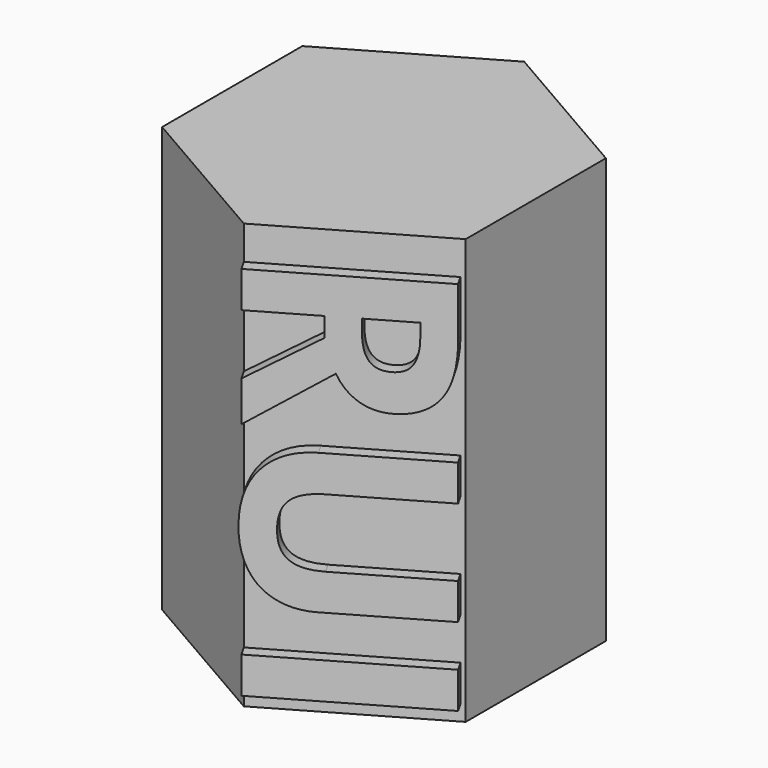
from build123d import *

# Parameters (mm, degrees)
F1_DEPTH     = 350
F3_TEXT_SIZE = 197.4233351479
F4_DEPTH     = 10
F6_DEPTH     = 300
F7_R         = 15


# Not quite as in the source:
# - Text() gives the source's letters only with a copy of the font that has no kerning and outlines rounded to 1/6400 em; it was checked with that copy


with BuildPart() as f1:
    # F0 (on Top) → F1 (new body)
    with BuildSketch(Plane.XY):
        Polygon((125, -72.1687836487), (125, 72.1687836487), (0, 144.3375672974), (-125, 72.1687836487), (-125, -72.1687836487), (0, -144.3375672974), align=None)
    extrude(amount=F1_DEPTH)

    # F3 (on face) → F4 (join)
    with BuildSketch(Plane(origin=(62.5, -108.2531754731, 0), x_dir=(0.8660254038, 0.5, 0), z_dir=(0.5, -0.8660254038, 0))):
        with Locations(Location((-72.1687836487, 340), (0, 0, -90))):
            Text('RUI', F3_TEXT_SIZE, font='Open Sans', font_style=FontStyle.BOLD, text_align=(TextAlign.LEFT, TextAlign.BOTTOM))
    extrude(amount=F4_DEPTH)

    # F5 (on face) → F6 (cut)
    with BuildSketch(Plane(origin=(0, 0, 0), x_dir=(1, 0, 0), z_dir=(0, 0, -1))):
        Polygon((-95.1994684166, -52.1636714464), (-2.4246695811, -108.5269937987), (92.7747988355, -56.3633223523), (95.1994684166, 52.1636714464), (2.4246695811, 108.5269937987), (-92.7747988355, 56.3633223523), align=None)
    extrude(amount=-F6_DEPTH, mode=Mode.SUBTRACT)

    # F10: sweep along a path in F9
    with BuildLine(Plane(origin=(0, 0, 0), x_dir=(-0.5, 0.8660254038, 0), z_dir=(0.8660254038, 0.5, 0))) as f10_path:
        ThreePointArc((121.8484041474, 50), (246.8484041474, 175), (121.8484041474, 300))
    # F7 (on face) → F10 (sweep)
    with BuildSketch(Plane(origin=(-62.5, 108.2531754731, 0), x_dir=(-0.8660254038, -0.5, 0), z_dir=(-0.5, 0.8660254038, 0))):
        with Locations((0, 50)):
            Circle(F7_R)
        with Locations((0, 300)):
            Circle(F7_R)
    sweep(path=f10_path.line)


solid = f1.part
